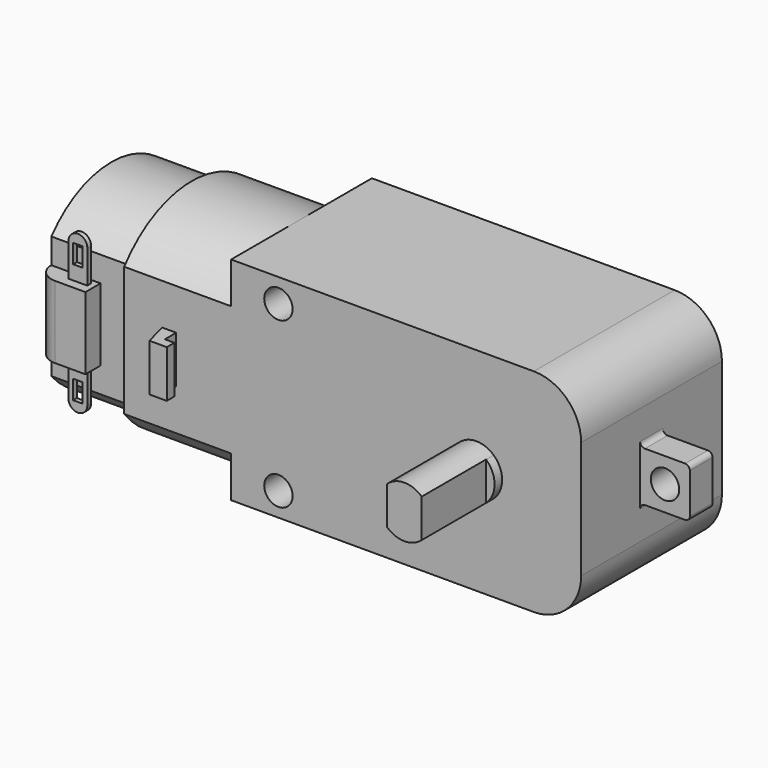
from build123d import *
from build123d import SkipClean  # not in build123d's __all__

# Parameters (mm, degrees)
F0_W           = 37
F0_H           = 18.6
F1_DEPTH       = 22.4
F3_DEPTH       = 11.3
F5_DEPTH       = 8.5
F7_DEPTH       = 2
F8_R           = 1
F9_DEPTH       = 1
F10_R          = 3.575
F11_DEPTH      = 0.5
F11_DEPTH_BACK = 19.1
F13_DEPTH      = 9
F13_DEPTH_BACK = 28.6
F14_R          = 5
F16_START      = -7.8
F15_W          = 5.25
F15_H          = 5.25
F15_R          = 1.5
F16_DEPTH      = 3
F17_R          = 0.5
F19_START      = -8.7
F19_DEPTH      = 5
F20_R          = 2
F21_DEPTH      = 2
F22_R          = 1.5
F23_DEPTH      = 28.101
F24_DEPTH      = 0.5
F25_R          = 2.725
F26_DEPTH      = 1
F26_DEPTH_BACK = 19.6
F27_W          = 5.2
F27_H          = 7.65
F28_DEPTH      = 2
F29_R          = 2
F31_START      = -1
F30_W          = 1
F30_H          = 2
F31_DEPTH      = 0.5


# Not quite as in the source:
# - after a boolean that leaves OpenCascade's solid faulty, fix() repairs it


with BuildPart() as f1:
    # F0 (on Top) → F1 (new body)
    with BuildSketch(Plane.XY):
        Rectangle(F0_W, F0_H)
    extrude(amount=F1_DEPTH)

    # F2 (on face) → F3 (join)
    with BuildSketch(Plane(origin=(-18.5, 0, 0), x_dir=(0, -1, 0), z_dir=(-1, 0, 0))):
        with BuildLine():
            ThreePointArc((-8.55, 4.35), (0.375, 0), (9.3, 4.35))
            Line((9.3, 4.35), (9.3, 18.05))
            ThreePointArc((9.3, 18.05), (0.375, 22.4), (-8.55, 18.05))
            Line((-8.55, 18.05), (-8.55, 4.35))
        make_face()
    extrude(amount=F3_DEPTH)

    # F4 (on face) → F5 (join)
    with BuildSketch(Plane(origin=(-29.8, 0, 0), x_dir=(0, -1, 0), z_dir=(-1, 0, 0))):
        with BuildLine():
            Line((-7.55, 17.6964123944), (-7.55, 4.7035876056))
            ThreePointArc((-7.55, 4.7035876056), (0.375, 1), (8.3, 4.7035876056))
            Line((8.3, 4.7035876056), (8.3, 17.6964123944))
            ThreePointArc((8.3, 17.6964123944), (0.375, 21.4), (-7.55, 17.6964123944))
        make_face()
    extrude(amount=F5_DEPTH)

    # F6 (on face) → F7 (join)
    with BuildSketch(Plane(origin=(-38.3, 0, 0), x_dir=(0, -1, 0), z_dir=(-1, 0, 0))):
        with BuildLine():
            Line((-3.525, 14.1664793948), (-3.525, 8.2335206052))
            ThreePointArc((-3.525, 8.2335206052), (5.275, 11.2), (-3.525, 14.1664793948))
        make_face()
    extrude(amount=F7_DEPTH)

    # F8 (on face) → F9 (join)
    with BuildSketch(Plane(origin=(-40.3, 0, 0), x_dir=(0, -1, 0), z_dir=(-1, 0, 0))):
        with Locations((0.375, 11.2)):
            Circle(F8_R)
    extrude(amount=F9_DEPTH)

    # F10 (on face) → F11 (join, two sides)
    with BuildSketch(Plane(origin=(0, 9.3, 0), x_dir=(-1, 0, 0), z_dir=(0, 1, 0))) as f11_sk:
        with Locations((-7.425, 11.2)):
            Circle(F10_R)
    extrude(amount=F11_DEPTH)
    extrude(f11_sk.sketch, amount=-F11_DEPTH_BACK)

    # F12 (on face) → F13 (join, two sides)
    with BuildSketch(Plane(origin=(0, 9.8, 0), x_dir=(-1, 0, 0), z_dir=(0, 1, 0))) as f13_sk:
        with BuildLine():
            Line((-5.6, 9.1763893655), (-5.6, 13.2236106345))
            ThreePointArc((-5.6, 13.2236106345), (-7.425, 13.925), (-9.25, 13.2236106345))
            Line((-9.25, 13.2236106345), (-9.25, 9.1763893655))
            ThreePointArc((-9.25, 9.1763893655), (-7.425, 8.475), (-5.6, 9.1763893655))
        make_face()
    extrude(amount=F13_DEPTH)
    extrude(f13_sk.sketch, amount=-F13_DEPTH_BACK)

    # F14
    f14_edges = [f1.edges().sort_by_distance(p)[0] for p in [
        (18.5, 0, 0),
        (18.5, 0, 22.4),
    ]]
    fillet(f14_edges, radius=F14_R)

    # F15 (on face) → F16 (join)
    with BuildSketch(Plane(origin=(0, 9.3, 0), x_dir=(-1, 0, 0), z_dir=(0, 1, 0)).offset(F16_START)):
        with Locations((-21.125, 11.2)):
            Rectangle(F15_W, F15_H)
        with Locations((-21.125, 11.2)):
            Circle(F15_R, mode=Mode.SUBTRACT)
    extrude(amount=-F16_DEPTH)

    # F17
    f17_edges = [f1.edges().sort_by_distance(p)[0] for p in [
        (23.75, 0, 13.825),
        (18.5, 0, 13.825),
        (23.75, 0, 8.575),
        (18.5, 0, 8.575),
    ]]
    fillet(f17_edges, radius=F17_R)

    # F18 (on face) → F19 (join)
    with BuildSketch(Plane.XY.offset(22.4).offset(F19_START)):
        Polygon((-25.1301270189, 11.05), (-25.8, 8.55), (-24.3, 8.55), (-24.3, 10.05), (-23.3, 10.05), (-23.3, 11.05), align=None)
        Polygon((-23.3, -10.8), (-24.3, -10.8), (-24.3, -9.3), (-25.8, -9.3), (-25.1301270189, -11.8), (-23.3, -11.8), align=None)
    extrude(amount=-F19_DEPTH)

    # F20 (on face) → F21 (join)
    with BuildSketch(Plane(origin=(0, 9.3, 0), x_dir=(-1, 0, 0), z_dir=(0, 1, 0))):
        with Locations((4, 11.2)):
            Circle(F20_R)
    extrude(amount=F21_DEPTH)

    # F22 (on face) → F23 (cut, through all)
    with BuildSketch(Plane(origin=(0, 9.3, 0), x_dir=(-1, 0, 0), z_dir=(0, 1, 0))):
        with Locations((13.5, 19.9)):
            Circle(F22_R)
        with Locations((13.5, 2.5)):
            Circle(F22_R)
    extrude(amount=-F23_DEPTH, mode=Mode.SUBTRACT)

    # F24 (cut): a face of the model
    f24_faces = [f1.faces().sort_by_distance(p)[0] for p in [
        (10.8988837303, -9.8, 11.2),
    ]]
    extrude(f24_faces, amount=-F24_DEPTH, mode=Mode.SUBTRACT)

    # F25 (on face) → F26 (join, two sides)
    with BuildSketch(Plane.XZ.offset(9.3)) as f26_sk:
        with Locations((7.425, 11.2)):
            Circle(F25_R)
    with SkipClean():  # cleaning this boolean's faces spoils the solid; the shape is the same uncleaned
        extrude(amount=F26_DEPTH)
        extrude(f26_sk.sketch, amount=-F26_DEPTH_BACK)

    # F27 (on face) → F28 (join)
    with BuildSketch(Plane.XZ.offset(8.3)):
        with Locations((-35.7, 11.2)):
            Rectangle(F27_W, F27_H)
    extrude(amount=F28_DEPTH)

    add(f1.part.fix(), mode=Mode.REPLACE)

    # F29
    f29_edges = [f1.edges().sort_by_distance(p)[0] for p in [
        (-38.3, -10.3, 11.2),
    ]]
    fillet(f29_edges, radius=F29_R)

    # F30 (on face) → F31 (join)
    with BuildSketch(Plane.XZ.offset(10.3).offset(F31_START)):
        with BuildLine():
            Line((-35.7, 18.525), (-35.7, 15.025))
            Line((-35.7, 15.025), (-33.7, 15.025))
            Line((-33.7, 15.025), (-33.7, 18.525))
            ThreePointArc((-33.7, 18.525), (-34.7, 19.525), (-35.7, 18.525))
        make_face()
        with Locations((-34.7, 17.525)):
            Rectangle(F30_W, F30_H, mode=Mode.SUBTRACT)
        with BuildLine():
            Line((-35.7, 7.375), (-35.7, 3.875))
            ThreePointArc((-35.7, 3.875), (-34.7, 2.875), (-33.7, 3.875))
            Line((-33.7, 3.875), (-33.7, 7.375))
            Line((-33.7, 7.375), (-35.7, 7.375))
        make_face()
        with Locations((-34.7, 4.875)):
            Rectangle(F30_W, F30_H, mode=Mode.SUBTRACT)
    extrude(amount=-F31_DEPTH)


solid = f1.part
